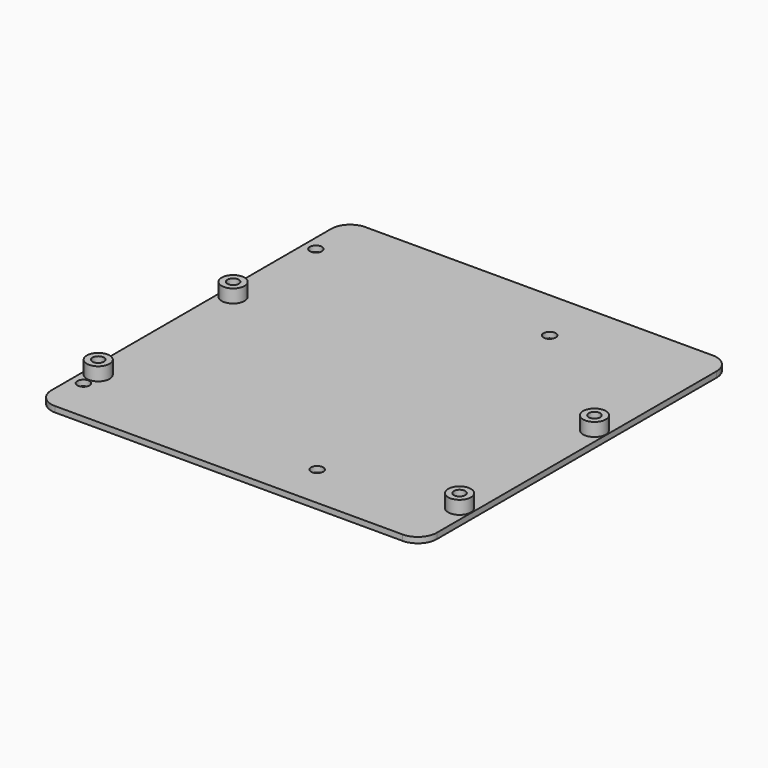
from build123d import *

# Parameters (mm, degrees)
F0_W     = 101.6
F0_H     = 147
F0_R     = 3
F1_DEPTH = 1.5
F2_R     = 1.6
F3_DEPTH = 25
F4_DEPTH = 5
F5_R     = 1.5
F6_DEPTH = 3
F7_W     = 101.6
F7_H     = 44.8
F8_DEPTH = 25
F9_R     = 5


# Not quite as in the source:
# - a feature names something its author has since deleted; it is built from what else it names


with BuildPart() as f1:
    # F0 (on Top) → F1 (new body)
    with BuildSketch(Plane.XY):
        with Locations((-19.733554095, 37.0265730321)):
            Rectangle(F0_W, F0_H)
        with Locations((-67.358554095, 24.7965730321)):
            Circle(F0_R, mode=Mode.SUBTRACT)
        with Locations((27.891445905, 24.7965730321)):
            Circle(F0_R, mode=Mode.SUBTRACT)
        with Locations((-67.358554095, 69.2465730321)):
            Circle(F0_R, mode=Mode.SUBTRACT)
        with Locations((27.891445905, 69.2465730321)):
            Circle(F0_R, mode=Mode.SUBTRACT)
    extrude(amount=F1_DEPTH)

    # F2 (on face) → F3 (cut)
    with BuildSketch(Plane.XY.offset(1.5)):
        with Locations((-67.358554095, 96.5265730321)):
            Circle(F2_R)
        with Locations((-5.758554095, 96.5265730321)):
            Circle(F2_R)
        with Locations((-67.358554095, 19.9265730321)):
            Circle(F2_R)
        with Locations((-5.758554095, 19.9265730321)):
            Circle(F2_R)
    extrude(amount=-F3_DEPTH, mode=Mode.SUBTRACT)

    # F0 (on Top) → F4 (join)
    with BuildSketch(Plane.XY):
        with Locations((-67.358554095, 69.2465730321)):
            Circle(F0_R)
        with Locations((-67.358554095, 24.7965730321)):
            Circle(F0_R)
        with Locations((27.891445905, 69.2465730321)):
            Circle(F0_R)
        with Locations((27.891445905, 24.7965730321)):
            Circle(F0_R)
    extrude(amount=F4_DEPTH)

    # F5 (on face) → F6 (cut)
    with BuildSketch(Plane.XY.offset(5)):
        with Locations((-67.358554095, 69.2465730321)):
            Circle(F5_R)
        with Locations((-67.358554095, 24.7965730321)):
            Circle(F5_R)
        with Locations((27.891445905, 69.2465730321)):
            Circle(F5_R)
        with Locations((27.891445905, 24.7965730321)):
            Circle(F5_R)
    extrude(amount=-F6_DEPTH, mode=Mode.SUBTRACT)

    # F7 (on face) → F8 (cut)
    with BuildSketch(Plane.XY.offset(1.5)):
        with Locations((-19.733554095, -14.0734269679)):
            Rectangle(F7_W, F7_H)
        Polygon((-70.533554095, 8.3265730321), (-108.6030122084, 8.3265730321), (-108.6030122084, -69.3553299345), (74.6913593453, -69.3553299345), (74.6913593453, 8.3265730321), (31.066445905, 8.3265730321), (31.066445905, -36.4734269679), (-70.533554095, -36.4734269679), align=None)
        Polygon((-108.166599336, 100.5265730321), (-70.533554095, 100.5265730321), (-70.533554095, 110.5265730321), (31.066445905, 110.5265730321), (31.066445905, 100.5265730321), (58.5440034669, 100.5265730321), (58.5440034669, 119.7288488672), (-108.166599336, 119.7288488672), align=None)
    extrude(amount=-F8_DEPTH, mode=Mode.SUBTRACT)

    # F9
    f9_edges = [f1.edges().sort_by_distance(p)[0] for p in [
        (-70.533554, 8.326573, 0.75),
        (-70.533554, 110.526573, 0.75),
        (31.066446, 8.326573, 0.75),
        (31.066446, 110.526573, 0.75),
    ]]
    fillet(f9_edges, radius=F9_R)


solid = f1.part
